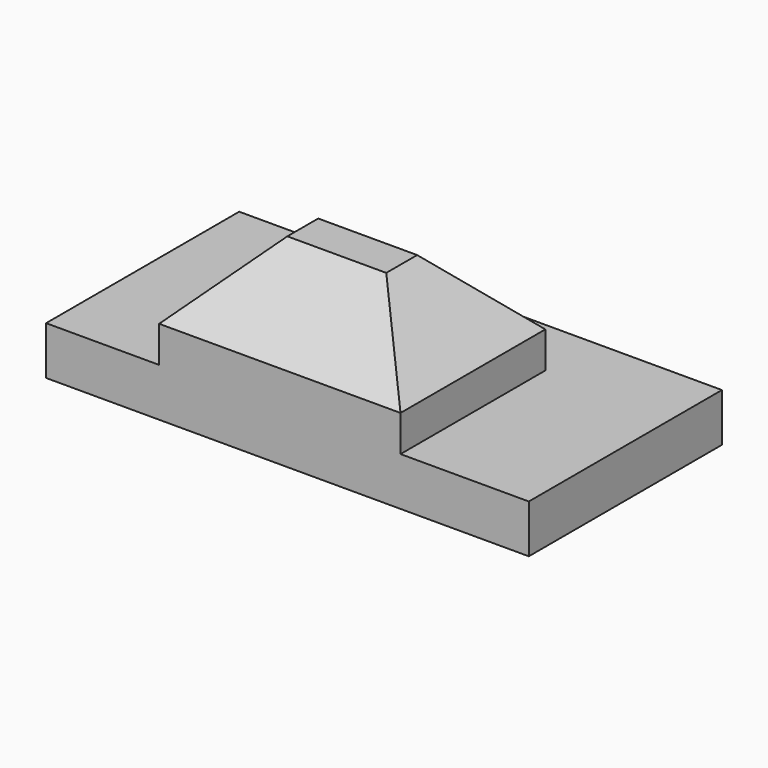
from build123d import *

# Parameters (mm, degrees)
F0_W      = 1016
F0_H      = 508
F1_DEPTH  = 101.6
F4_W      = 237.9516797066
F4_H      = 381
F4_W_2    = 270.0483202934
F5_DEPTH  = 76.2
F5_FACE_W = 508
F5_FACE_H = 381
F6_DEPTH  = 149.86
F6_TAPER  = 45
F7_R      = 63.5
F8_DEPTH  = 76.2


# Not quite as in the source:
# - the program builds the solid bodies; features that only make, move or delete a surface that nothing else refers to are left out


with BuildPart() as f1:
    # F0 (on Top) → F1 (new body)
    with BuildSketch(Plane.XY):
        Rectangle(F0_W, F0_H)
    extrude(amount=F1_DEPTH)

    # F4 (on face) → F5 (join)
    with BuildSketch(Plane.XY.offset(101.6)):
        with Locations((118.9758398533, -63.5)):
            Rectangle(F4_W, F4_H)
        with Locations((-135.0241601467, -63.5)):
            Rectangle(F4_W_2, F4_H)
    extrude(amount=F5_DEPTH)

    # F5_face (on face) → F6 (join, symmetric)
    with BuildSketch(Plane(origin=(-16.0483202934, -63.5, 177.8), x_dir=(1, 0, 0), z_dir=(0, 0, 1))):
        Rectangle(F5_FACE_W, F5_FACE_H)
    extrude(amount=F6_DEPTH, both=True, taper=F6_TAPER)

    # F7 (on face) → F8 (cut)
    with BuildSketch(Plane(origin=(0, 152.4, 152.4), x_dir=(-1, 0, 0), z_dir=(0, 0.7071067812, 0.7071067812))):
        with Locations((10.2272699534, 145.9400733915)):
            Circle(F7_R)
    extrude(amount=-F8_DEPTH, mode=Mode.SUBTRACT)


solid = f1.part
